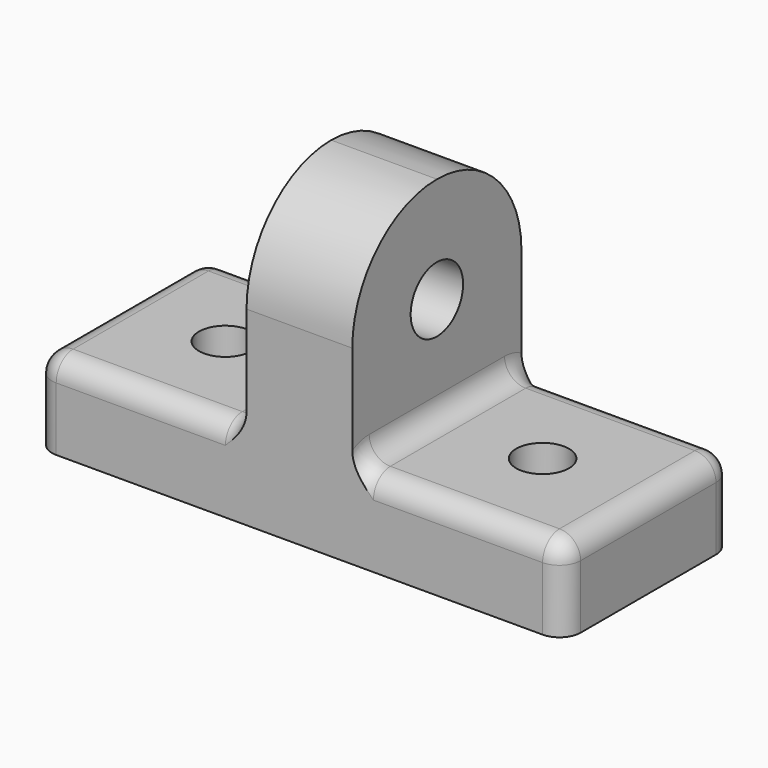
from build123d import *

# Parameters (mm, degrees)
F0_W          = 25
F0_H          = 10
F1_DEPTH      = 4
F2_W          = 5
F2_H          = 10
F3_DEPTH      = 10
F4_R          = 1.25
F5_DEPTH      = 4.001
F7_R          = 4.99999
F8_R          = 1.55
F9_DEPTH      = 15.001
F10_R         = 1
F11_T1_DEPTH  = 8
F11_T6_ANGLE  = 233.2969892374
F11_T11_ANGLE = 233.2969892374
F11_T16_ANGLE = 233.2969892374
F11_T21_ANGLE = 233.2969892374


# Not quite as in the source:
# - a fillet or chamfer that OpenCascade refuses, or shapes differently, is made with other operations: its cross-section is extruded or revolved along the edge and cut away or added
# - a fillet or chamfer is up to 0.001 mm smaller than in the source, because OpenCascade refuses the exact size
# - a pattern or mirror of a feature is missing from the dataset's text; its kind, count and spacing are read off the source's solid


with BuildPart() as f1:
    # F0 (on Top) → F1 (new body)
    with BuildSketch(Plane.XY):
        Rectangle(F0_W, F0_H)
    extrude(amount=F1_DEPTH)

    # F2 (on face) → F3 (join)
    with BuildSketch(Plane.XY.offset(4)):
        Rectangle(F2_W, F2_H)
    extrude(amount=F3_DEPTH)

    # F4 (on face) → F5 (cut, through all)
    with BuildSketch(Plane.XY.offset(4)):
        with Locations((-7.5, 0)):
            Circle(F4_R)
    f5 = extrude(amount=-F5_DEPTH, mode=Mode.SUBTRACT)

    # F5_copies: F5 across plane
    add(f5.mirror(Plane(origin=(0, 0, 0), x_dir=(0, 0, 1), z_dir=(1, 0, 0))), mode=Mode.SUBTRACT)

    # F7 (radius 5 in the source; OpenCascade refuses exactly that, so slightly less here)
    f7_edges = [f1.edges().sort_by_distance(p)[0] for p in [
        (0, -5, 14),
        (0, 5, 14),
    ]]
    fillet(f7_edges, radius=F7_R)

    # F8 (on face) → F9 (cut, through all)
    with BuildSketch(Plane(origin=(-2.5, 0, 0), x_dir=(0, -1, 0), z_dir=(-1, 0, 0))):
        with Locations((0, 9)):
            Circle(F8_R)
    extrude(amount=-F9_DEPTH, mode=Mode.SUBTRACT)

    # F10
    f10_edges = [f1.edges().sort_by_distance(p)[0] for p in [
        (7.5, -5, 4),
        (12.5, 0, 4),
        (7.5, 5, 4),
        (12.5, -5, 2),
        (12.5, 5, 2),
        (-12.5, -5, 2),
        (-12.5, 5, 2),
        (-12.5, 0, 4),
        (-7.5, -5, 4),
        (-7.5, 5, 4),
    ]]
    fillet(f10_edges, radius=F10_R)

    # F11: fillet of radius 1 on 2 edges, made by hand

    # F11_s2 → F11_t1 (join)
    with BuildSketch(Plane.XZ.offset(-4)):
        with BuildLine():
            ThreePointArc((2.5, 5), (2.7928932188, 4.2928932188), (3.5, 4))
            Line((3.5, 4), (2.5, 4))
            Line((2.5, 4), (2.5, 5))
        make_face()
        with BuildLine():
            ThreePointArc((-2.5, 5), (-2.7928932188, 4.2928932188), (-3.5, 4))
            Line((-3.5, 4), (-2.5, 4))
            Line((-2.5, 4), (-2.5, 5))
        make_face()
    extrude(amount=F11_T1_DEPTH)


with BuildPart() as f11_tool4:
    # F11_s5 → F11_t6 (revolve)
    with BuildSketch(Plane.XZ.offset(-4)):
        with BuildLine():
            ThreePointArc((-2.5, 5), (-2.7928932188, 4.2928932188), (-3.5, 4))
            Line((-3.5, 4), (-2.5, 4))
            Line((-2.5, 4), (-2.5, 5))
        make_face()
    revolve(axis=Axis((-2.5, 4, 3), (-1, 0, 0)), revolution_arc=F11_T6_ANGLE)

    split(bisect_by=Plane.XZ.offset(-5), keep=Keep.TOP)


with BuildPart() as f1_1:
    add(f1.part)

    # F11_t3: union F11_tool4
    add(f11_tool4.part)


with BuildPart() as f11_tool9:
    # F11_s10 → F11_t11 (revolve)
    with BuildSketch(Plane(origin=(0, 0.0087041916, 0.0116762883), x_dir=(1, 0, 0), z_dir=(0, 0.5976672776, 0.8017442393))):
        with BuildLine():
            ThreePointArc((-3.5, -3.9999787901), (-2.7928932188, -3.7070855713), (-2.5, -2.9999787901))
            Line((-2.5, -2.9999787901), (-2.5, -3.9999787901))
            Line((-2.5, -3.9999787901), (-3.5, -3.9999787901))
        make_face()
    revolve(axis=Axis((-2.5, -4, 3), (-1, 0, 0)), revolution_arc=F11_T11_ANGLE)

    split(bisect_by=Plane.XZ.offset(5), keep=Keep.BOTTOM)


with BuildPart() as f1_2:
    add(f1_1.part)

    # F11_t8: union F11_tool9
    add(f11_tool9.part)


with BuildPart() as f11_tool14:
    # F11_s15 → F11_t16 (revolve)
    with BuildSketch(Plane(origin=(0, 0.0087041916, 0.0116762883), x_dir=(1, 0, 0), z_dir=(0, 0.5976672776, 0.8017442393))):
        with BuildLine():
            ThreePointArc((3.5, -3.9999787901), (2.7928932188, -3.7070855713), (2.5, -2.9999787901))
            Line((2.5, -2.9999787901), (2.5, -3.9999787901))
            Line((2.5, -3.9999787901), (3.5, -3.9999787901))
        make_face()
    revolve(axis=Axis((2.5, -4, 3), (-1, 0, 0)), revolution_arc=F11_T16_ANGLE)

    split(bisect_by=Plane.XZ.offset(5), keep=Keep.BOTTOM)


with BuildPart() as f1_3:
    add(f1_2.part)

    # F11_t13: union F11_tool14
    add(f11_tool14.part)


with BuildPart() as f11_tool19:
    # F11_s20 → F11_t21 (revolve)
    with BuildSketch(Plane.XZ.offset(-4)):
        with BuildLine():
            ThreePointArc((2.5, 5), (2.7928932188, 4.2928932188), (3.5, 4))
            Line((3.5, 4), (2.5, 4))
            Line((2.5, 4), (2.5, 5))
        make_face()
    revolve(axis=Axis((2.5, 4, 3), (-1, 0, 0)), revolution_arc=F11_T21_ANGLE)

    split(bisect_by=Plane.XZ.offset(-5), keep=Keep.TOP)


with BuildPart() as f1_4:
    add(f1_3.part)

    # F11_t18: union F11_tool19
    add(f11_tool19.part)


solid = f1_4.part
